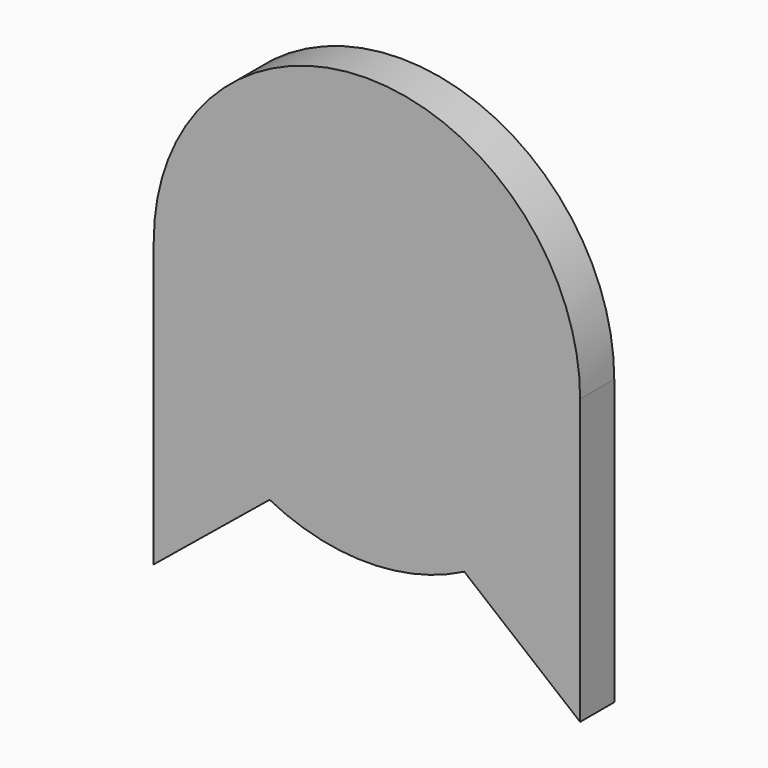
from build123d import *

# Parameters (mm, degrees)
F1_DEPTH = 15.24


# Not quite as in the source:
# - a feature names something its author has since deleted; it is built from what else it names


with BuildPart() as f1:
    # F0 (on Front) → F1 (new body)
    with BuildSketch(Plane.XZ):
        with BuildLine():
            ThreePointArc((34.7869106265, -67.7960975946), (65.0276963676, -39.7220178884), (76.2, 0))
            ThreePointArc((76.2, 0), (0, 76.2), (-76.2, 0))
            ThreePointArc((-76.2, 0), (-65.0276963676, -39.7220178884), (-34.7869106265, -67.7960975946))
            ThreePointArc((-34.7869106265, -67.7960975946), (0, -76.2), (34.7869106265, -67.7960975946))
        make_face()
        with BuildLine():
            Line((76.2, -101.6), (76.2, 0))
            ThreePointArc((76.2, 0), (65.0276963676, -39.7220178884), (34.7869106265, -67.7960975946))
            Line((34.7869106265, -67.7960975946), (76.2, -101.6))
        make_face()
        with BuildLine():
            ThreePointArc((-34.7869106265, -67.7960975946), (-65.0276963676, -39.7220178884), (-76.2, 0))
            Line((-76.2, 0), (-76.2, -101.6))
            Line((-76.2, -101.6), (-34.7869106265, -67.7960975946))
        make_face()
    extrude(amount=F1_DEPTH)


solid = f1.part
